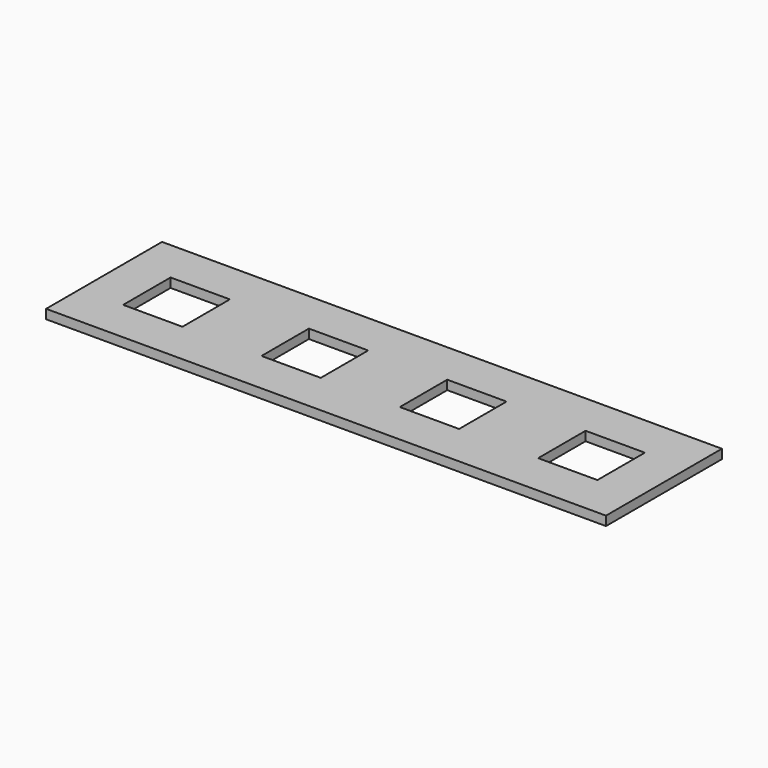
from build123d import *

# Parameters (mm, degrees)
F0_W     = 410
F0_H     = 110
F1_DEPTH = 7
F2_W     = 45
F2_H     = 45
F3_DEPTH = 25
F0_W_2   = 15
F4_DEPTH = 7


# Not quite as in the source:
# - a feature names something its author has since deleted; it is built from what else it names


with BuildPart() as f1:
    # F0 (on Top) → F1 (new body)
    with BuildSketch(Plane.XY):
        Rectangle(F0_W, F0_H)
    extrude(amount=F1_DEPTH)

    # F2 (on face) → F3 (cut)
    with BuildSketch(Plane.XY.offset(7)):
        with Locations((-60, 0)):
            Rectangle(F2_W, F2_H)
        with Locations((45, 0)):
            Rectangle(F2_W, F2_H)
        with Locations((150, 0)):
            Rectangle(F2_W, F2_H)
        with Locations((-165, 0)):
            Rectangle(F2_W, F2_H)
    extrude(amount=-F3_DEPTH, mode=Mode.SUBTRACT)

    # F0 (on Top) → F4 (join)
    with BuildSketch(Plane.XY):
        with Locations((-212.5, 0)):
            Rectangle(F0_W_2, F0_H)
    extrude(amount=F4_DEPTH)


solid = f1.part
